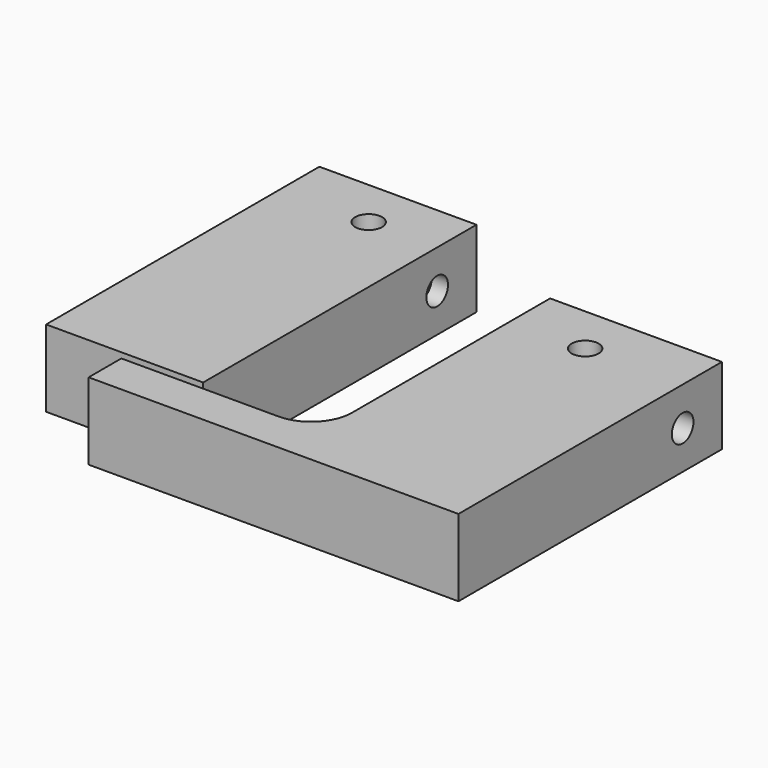
from build123d import *

# Parameters (mm, degrees)
F1_DEPTH  = 3.4
F3_DEPTH  = 3
F4_DEPTH  = 3
F5_DEPTH  = 3
F6_R      = 1.65
F7_DEPTH  = 3
F8_R      = 1.65
F9_DEPTH  = 2
F10_R     = 1.65
F11_DEPTH = 21.001
F12_R     = 5


# Not quite as in the source:
# - a feature names something its author has since deleted; it is built from what else it names


with BuildPart() as f1:
    # F0 (on Top) → F1 (new body)
    with BuildSketch(Plane.XY):
        Polygon((-17.2, 0), (0, 0), (-7, 3.75), (-14.2, 35.25), (-14.2, 40.75), (-17.2, 40.75), align=None)
        Polygon((0, 40.75), (0, 0), (-17.2, 0), (-17.2, -1), (2, -1), (2, 0), (2, 40.75), align=None)
    extrude(amount=F1_DEPTH)

    # F2 (on face) → F3 (join)
    with BuildSketch(Plane.XY.offset(3.4)):
        Polygon((0, 40.75), (0, 0), (-7, 3.75), (-14.2, 35.25), (-14.2, 40.75), (-17.2, 40.75), (-17.2, -1), (2, -1), (2, 0), (2, 40.75), align=None)
        Polygon((-7, 3.75), (0, 0), (0, 40.75), (-14.2, 40.75), (-14.2, 35.25), align=None)
    extrude(amount=F3_DEPTH)

    # F0 (on Top) → F4 (join)
    with BuildSketch(Plane.XY):
        Polygon((-17.2, 0), (0, 0), (-7, 3.75), (-14.2, 35.25), (-14.2, 40.75), (-17.2, 40.75), align=None)
        Polygon((-7, 3.75), (0, 0), (0, 40.75), (-14.2, 40.75), (-14.2, 35.25), align=None)
        Polygon((0, 40.75), (0, 0), (-17.2, 0), (-17.2, -1), (2, -1), (2, 0), (2, 40.75), align=None)
    extrude(amount=-F4_DEPTH)


with BuildPart() as f1b:
    # F0 (on Top) → F1, piece 2 (new body)
    with BuildSketch(Plane.XY):
        Polygon((20, 33.25), (17, 33.25), (17, 0), (17, -2), (-7.2, -2), (-7.2, -7), (38, -7), (38, 33.25), (33, 33.25), (27, 3.75), (20, 0), align=None)
    extrude(amount=F1_DEPTH)

    # F2 (on face) → F3, piece 2 (join)
    with BuildSketch(Plane.XY.offset(3.4)):
        Polygon((27, 3.75), (20, 0), (20, 33.25), (17, 33.25), (17, -2), (-7.2, -2), (-7.2, -7), (38, -7), (38, 33.25), (33, 33.25), align=None)
        Polygon((20, 33.25), (20, 0), (27, 3.75), (33, 33.25), align=None)
    extrude(amount=F3_DEPTH)

    # F0 (on Top) → F5 (join)
    with BuildSketch(Plane.XY):
        Polygon((20, 33.25), (17, 33.25), (17, 0), (17, -2), (-7.2, -2), (-7.2, -7), (38, -7), (38, 33.25), (33, 33.25), (27, 3.75), (20, 0), align=None)
        Polygon((33, 33.25), (20, 33.25), (20, 0), (27, 3.75), align=None)
    extrude(amount=-F5_DEPTH)


with BuildPart() as f7_tool:
    # F6 (on face) → F7 (new body, through all)
    with BuildSketch(Plane.XY.offset(6.4)):
        with Locations((-6.3778683543, 34.75)):
            Circle(F6_R)
        with Locations((26.0853748769, 27.25)):
            Circle(F6_R)
    extrude(amount=-F7_DEPTH)


with BuildPart() as f1_1:
    add(f1.part)

    # F7: cut by f7_tool
    add(f7_tool.part, mode=Mode.SUBTRACT)

    # F8 (on face) → F9 (cut, through all)
    with BuildSketch(Plane.YZ.offset(2)):
        with Locations((34.75, 1.7)):
            Circle(F8_R)
    extrude(amount=-F9_DEPTH, mode=Mode.SUBTRACT)


with BuildPart() as f1b_1:
    add(f1b.part)

    # F7: cut by f7_tool
    add(f7_tool.part, mode=Mode.SUBTRACT)

    # F10 (on face) → F11 (cut, through all)
    with BuildSketch(Plane(origin=(17, 0, 0), x_dir=(0, -1, 0), z_dir=(-1, 0, 0))):
        with Locations((-27.25, 1.7)):
            Circle(F10_R)
    extrude(amount=-F11_DEPTH, mode=Mode.SUBTRACT)

    # F12
    f12_edges = [f1b_1.edges().sort_by_distance(p)[0] for p in [
        (17, -2, 1.7),
    ]]
    fillet(f12_edges, radius=F12_R)


solid = Compound([f1_1.part, f1b_1.part])
